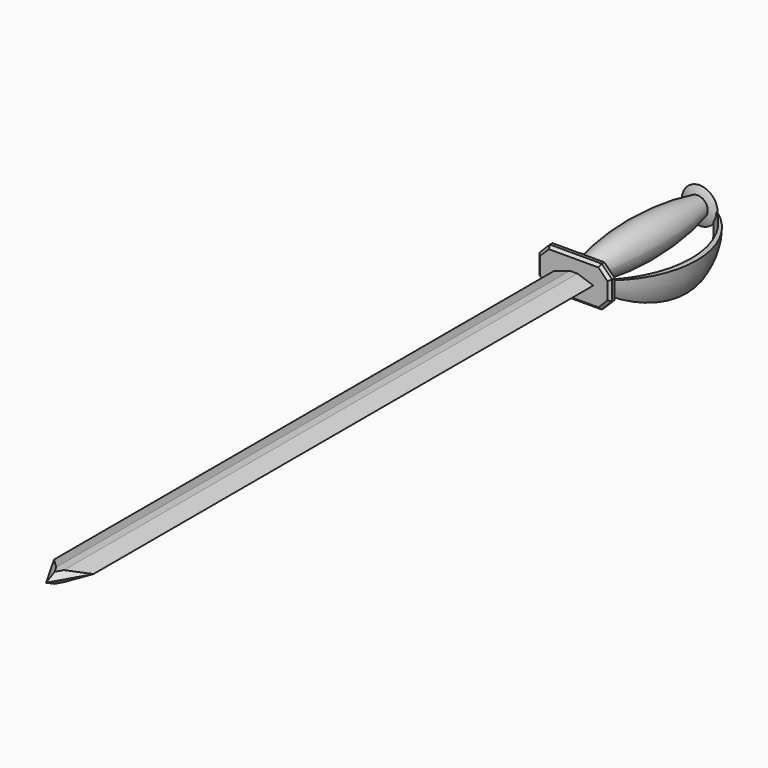
from build123d import *

# Parameters (mm, degrees)
F5_ANGLE     = 35
F6_R         = 8.5102699217
F6_R_2       = 4.6622389928
F7_DEPTH     = 0.762
F8_W         = 35.0466817617
F8_H         = 19.4376930594
F8_R         = 8.5102699217
F9_DEPTH     = 4.064
F10_SIZE     = 5.08
F11_SIZE     = 1.27
F12_W        = 18.9497359097
F12_H        = 5.1134214737
F13_DEPTH    = 320.04
F14_SIZE2    = 7.61999
F14_SIZE     = 2.556703
F14_2_SIZE2  = 7.61999
F14_2_SIZE   = 2.556703
F16_DEPTH    = 25.4
F17_T1_DEPTH = 30.0464510696
F17_T3_DEPTH = 30.0464510696


# Not quite as in the source:
# - a fillet or chamfer that OpenCascade refuses, or shapes differently, is made with other operations: its cross-section is extruded or revolved along the edge and cut away or added
# - a fillet or chamfer is up to 0.001 mm smaller than in the source, because OpenCascade refuses the exact size


with BuildPart() as f1:
    # F0 (on Top) → F1 (revolve)
    with BuildSketch(Plane.XY):
        with BuildLine():
            Line((0, 37.1474996209), (0, -33.8388159871))
            Line((0, -33.8388159871), (4.6622389928, -33.8388159871))
            ThreePointArc((4.6622389928, -33.8388159871), (8.7518845263, 1.6543418169), (4.6622389928, 37.1474996209))
            Line((4.6622389928, 37.1474996209), (0, 37.1474996209))
        make_face()
    revolve(axis=Axis((0, 1.6543418169, 0), (0, 1, 0)))


with BuildPart() as f3:
    # F2 (on Top) → F3 (revolve)
    with BuildSketch(Plane.XY):
        with BuildLine():
            Line((0, 38.9180295169), (0, 37.1474996209))
            Line((0, 37.1474996209), (0, 35.3769697249))
            ThreePointArc((0, 35.3769697249), (4.4347721966, 35.6315210034), (8.6101535708, 37.1474996209))
            ThreePointArc((8.6101535708, 37.1474996209), (4.4347721966, 38.6634782385), (0, 38.9180295169))
        make_face()
    revolve(axis=Axis((0, 38.0327645689, 0), (0, 1, 0)))

    # F4 (on Top) → F5 (revolve)
    with BuildSketch(Plane.XY):
        with BuildLine():
            Line((8.1650372595, 37.3600125313), (8.1650372595, 37.2307524085))
            Line((8.1650372595, 37.2307524085), (8.1650372595, 36.9532480836))
            ThreePointArc((8.1650372595, 36.9532480836), (24.4029578966, 1.5522614121), (8.1650372595, -33.8487252593))
            Line((8.1650372595, -33.8487252593), (8.1650372595, -34.227949133))
            ThreePointArc((8.1650372595, -34.227949133), (27.04288668, 1.5660316991), (8.1650372595, 37.3600125313))
        make_face()
    revolve(axis=Axis((0, 1.6543418169, 0), (0, 1, 0)), revolution_arc=F5_ANGLE)

    # F6 (on face) → F7 (join)
    with BuildSketch(Plane.XZ.offset(33.8388159871)):
        Circle(F6_R)
        Circle(F6_R_2, mode=Mode.SUBTRACT)
        Circle(F6_R_2)
    extrude(amount=F7_DEPTH)


with BuildPart() as f9:
    # F8 (on face) → F9 (new body)
    with BuildSketch(Plane.XZ.offset(34.6008159871)):
        Rectangle(F8_W, F8_H)
        Circle(F8_R, mode=Mode.SUBTRACT)
        Circle(F8_R)
    extrude(amount=F9_DEPTH)

    # F10
    f10_edges = [f9.edges().sort_by_distance(p)[0] for p in [
        (-17.523341, -36.632816, 9.718847),
        (-17.523341, -36.632816, -9.718847),
        (17.523341, -36.632816, 9.718847),
        (17.523341, -36.632816, -9.718847),
    ]]
    chamfer(f10_edges, length=F10_SIZE)

    # F11
    f11_edges = [f9.edges().sort_by_distance(p)[0] for p in [
        (17.523341, -38.664816, 0),
        (14.983341, -38.664816, -7.178847),
        (14.983341, -38.664816, 7.178847),
        (0, -38.664816, -9.718847),
        (0, -38.664816, 9.718847),
        (-14.983341, -38.664816, -7.178847),
        (-14.983341, -38.664816, 7.178847),
        (-17.523341, -38.664816, 0),
        (17.523341, -34.600816, 0),
        (14.983341, -34.600816, -7.178847),
        (14.983341, -34.600816, 7.178847),
        (0, -34.600816, -9.718847),
        (0, -34.600816, 9.718847),
        (-14.983341, -34.600816, -7.178847),
        (-14.983341, -34.600816, 7.178847),
        (-17.523341, -34.600816, 0),
    ]]
    chamfer(f11_edges, length=F11_SIZE)


with BuildPart() as f13:
    # F12 (on face) → F13 (new body)
    with BuildSketch(Plane.XZ.offset(38.6648159871)):
        Rectangle(F12_W, F12_H)
    extrude(amount=F13_DEPTH)

    # F14 (size 2.5567132 and 7.62 in the source; OpenCascade refuses exactly that, so slightly less here)
    f14_edges = [f13.edges().sort_by_distance(p)[0] for p in [
        (-9.474868, -198.684816, 2.556711),
        (-9.474868, -198.684816, -2.556711),
    ]]
    f14_side = f13.faces().sort_by_distance((-9.474868, -198.684816, 0))[0]
    chamfer(f14_edges, length=F14_SIZE, length2=F14_SIZE2, reference=f14_side)

    # F14#2 (size 2.5567132 and 7.62 in the source; OpenCascade refuses exactly that, so slightly less here)
    f14_2_edges = [f13.edges().sort_by_distance(p)[0] for p in [
        (9.474868, -198.684816, 2.556711),
        (9.474868, -198.684816, -2.556711),
    ]]
    f14_2_side = f13.faces().sort_by_distance((9.474868, -198.684816, 0))[0]
    chamfer(f14_2_edges, length=F14_2_SIZE, length2=F14_2_SIZE2, reference=f14_2_side)

    # F15 (on face) → F16 (cut)
    with BuildSketch(Plane.XY.offset(2.5567107368)):
        Polygon((11.3733373582, -335.993885994), (1.8548779549, -352.6961032261), (1.8548779549, -358.7048159871), (-1.8548779549, -358.7048159871), (-1.8548779549, -352.6961032261), (-11.3733373582, -335.993885994), (-10.944146663, -359.4379723072), (13.7874875218, -359.4379723072), align=None)
        Polygon((1.8548779549, -352.6961032261), (0, -355.9508919716), (-1.8548779549, -352.6961032261), (-1.8548779549, -358.7048159871), (1.8548779549, -358.7048159871), align=None)
    extrude(amount=-F16_DEPTH, mode=Mode.SUBTRACT)

    # F17: chamfer of 2.5567132 on 4 edges, made by hand

    # F17_s2 → F17_t1 (cut)
    with BuildSketch(Plane(origin=(156.378331212, -274.399957767, 0), x_dir=(0, 0, 1), z_dir=(-0.4951321974, 0.8688176489, 0))):
        Polygon((2.5567107368, -173.6860341202), (-2.4632e-06, -176.2427473202), (2.5567107368, -176.2427473202), align=None)
        Polygon((2.4632e-06, -176.2427473202), (-2.5567107368, -173.6860341202), (-2.5567107368, -176.2427473202), align=None)
    extrude(amount=F17_T1_DEPTH, mode=Mode.SUBTRACT)

    # F17_s4 → F17_t3 (cut)
    with BuildSketch(Plane(origin=(-141.5013658689, -248.2950707905, 0), x_dir=(0, 0, 1), z_dir=(-0.4951321974, -0.8688176489, 0))):
        Polygon((2.5567107368, -173.6860341202), (-2.4632e-06, -176.2427473202), (2.5567107368, -176.2427473202), align=None)
        Polygon((2.4632e-06, -176.2427473202), (-2.5567107368, -173.6860341202), (-2.5567107368, -176.2427473202), align=None)
    extrude(amount=F17_T3_DEPTH, mode=Mode.SUBTRACT)


solid = Compound([f1.part, f3.part, f9.part, f13.part])
